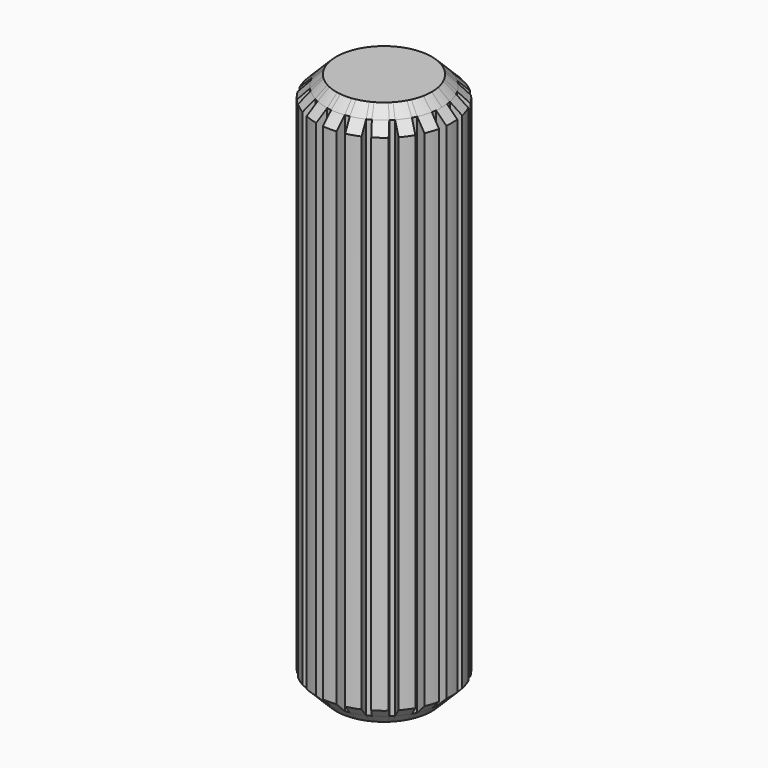
from build123d import *

# Parameters (mm, degrees)
F1_DEPTH = 20
F2_SIZE  = 0.75
F3_DEPTH = 19.25
F4_SIZE  = 0.74999
F5_COUNT = 20


# Not quite as in the source:
# - a fillet or chamfer is up to 0.001 mm smaller than in the source, because OpenCascade refuses the exact size


with BuildPart() as f1:
    # F0 (on Top) → F1 (new body, symmetric)
    with BuildSketch(Plane.XY):
        with BuildLine():
            ThreePointArc((4.25, 0), (3.1770662568, 2.8228974477), (0.5, 4.220485754))
            Line((0.5, 4.220485754), (0.5, 0))
            ThreePointArc((0.5, 0), (0, -0.5), (-0.5, 0))
            Line((-0.5, 0), (-0.5, 4.220485754))
            ThreePointArc((-0.5, 4.220485754), (-2.8228974477, -3.1770662568), (4.25, 0))
        make_face()
        with BuildLine():
            ThreePointArc((-0.5, 0), (0, -0.5), (0.5, 0))
            ThreePointArc((0.5, 0), (0, 0.5), (-0.5, 0))
        make_face()
        with BuildLine():
            Line((0.5, 0), (0.5, 4.220485754))
            ThreePointArc((0.5, 4.220485754), (0, 4.25), (-0.5, 4.220485754))
            Line((-0.5, 4.220485754), (-0.5, 0))
            ThreePointArc((-0.5, 0), (0, 0.5), (0.5, 0))
        make_face()
    extrude(amount=F1_DEPTH, both=True)

    # F2
    f2_edges = [f1.edges().sort_by_distance(p)[0] for p in [
        (-0.5, -4.220486, 20),
        (-0.5, -4.220486, -20),
    ]]
    chamfer(f2_edges, length=F2_SIZE)

    # F0 (on Top) → F3 (join, symmetric)
    with BuildSketch(Plane.XY):
        with BuildLine():
            Line((0.5, 4.220485754), (0.5, 4.9749371855))
            ThreePointArc((0.5, 4.9749371855), (0, 5), (-0.5, 4.9749371855))
            Line((-0.5, 4.9749371855), (-0.5, 4.220485754))
            ThreePointArc((-0.5, 4.220485754), (0, 4.25), (0.5, 4.220485754))
        make_face()
    extrude(amount=F3_DEPTH, both=True)

    # F4 (size 0.75 in the source; OpenCascade refuses exactly that, so slightly less here)
    f4_edges = [f1.edges().sort_by_distance(p)[0] for p in [
        (0, 5, 19.25),
        (0, 5, -19.25),
    ]]
    chamfer(f4_edges, length=F4_SIZE)

    # F5: F1 ×20 about axis
    f5_axis = Axis((0, 0, 0), (0, 0, 1))


with BuildPart() as f1_1:
    add(f1.part)
    for i in range(1, F5_COUNT):
        add(f1.part.rotate(f5_axis, i * 360 / F5_COUNT))


solid = f1_1.part
